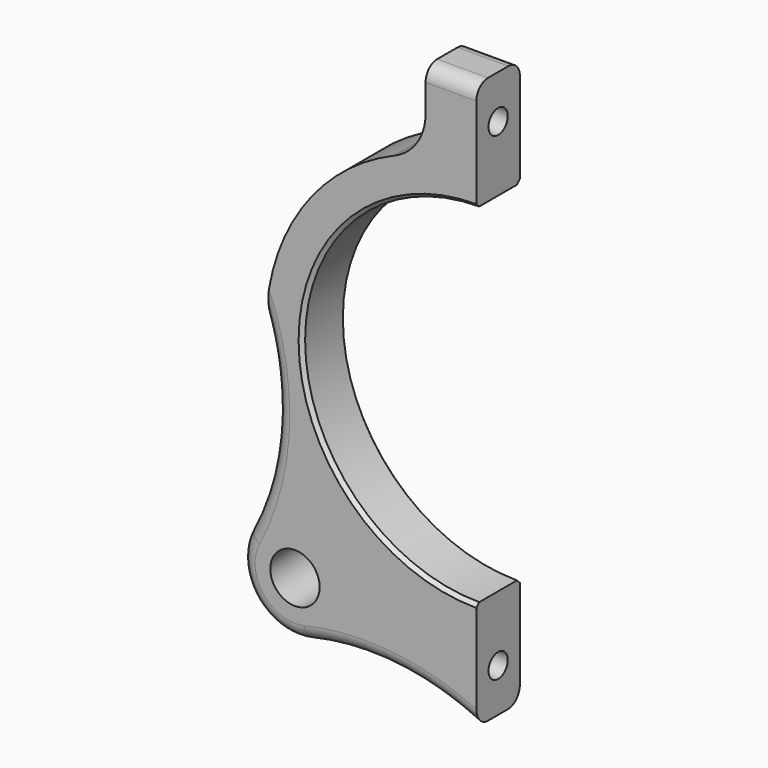
from build123d import *
from build123d import SkipClean  # not in build123d's __all__

# Parameters (mm, degrees)
F1_DEPTH    = 3.75
F3_D        = 3.3
F3_DEPTH    = 12.2
F3_TIP      = 0.9914200214
F4_R        = 2
F5_T4_DEPTH = 7.5
F5_S5_R     = 1.65
F5_T6_DEPTH = 7
F6_SIZE     = 0.5
F8_D        = 6.8


# Not quite as in the source:
# - a fillet or chamfer that OpenCascade refuses, or shapes differently, is made with other operations: its cross-section is extruded or revolved along the edge and cut away or added
# - a feature names something its author has since deleted; it is built from what else it names


with BuildPart() as f1:
    # F0 (on Front) → F1 (new body, symmetric)
    with BuildSketch(Plane.XZ):
        with BuildLine():
            ThreePointArc((0, -24), (-24, 0), (0, 24))
            Line((0, 24), (0, 39))
            Line((0, 39), (-7, 39))
            Line((-7, 39), (-7, 28.1424945589))
            ThreePointArc((-7, 28.1424945589), (-22.8473193176, 17.8605710995), (-29, 0))
            ThreePointArc((-29, 0), (-27.9004726433, -13.0232858743), (-31.6552133192, -25.541946259))
            ThreePointArc((-31.6552133192, -25.541946259), (-30.9284075442, -33.5939072683), (-23.3128108861, -36.3077625094))
            ThreePointArc((-23.3128108861, -36.3077625094), (-11.4240360348, -35.6417318474), (0, -39))
            Line((0, -39), (0, -24))
        make_face()
    extrude(amount=F1_DEPTH, both=True)

    # F3
    with Locations(Plane.YZ):
        with Locations((0, 33), (0, -33)):
            Hole(F3_D / 2, depth=F3_DEPTH)
            with Locations((0, 0, -(F3_DEPTH + F3_TIP / 2))):  # 118° drill point
                Cone(0, F3_D / 2, F3_TIP, mode=Mode.SUBTRACT)

    # F4
    f4_edges = [f1.edges().sort_by_distance(p)[0] for p in [
        (-3.5, 3.75, 39),
        (-3.5, -3.75, 39),
        (-11.424036, 3.75, -35.641732),
        (-11.424036, -3.75, -35.641732),
    ]]
    fillet(f4_edges, radius=F4_R)

    # F5: fillet of radius 7 on 1 edges, made by hand


with BuildPart() as f5_tool2:
    # F5_s3 → F5_t4 (new body)
    with BuildSketch(Plane.XZ.offset(-3.75)):
        with BuildLine():
            ThreePointArc((-11.2777777778, 26.7172552556), (-8.1666666667, 29.2968523148), (-7, 33.1662479036))
            Line((-7, 33.1662479036), (-7, 28.1424945589))
            ThreePointArc((-7, 28.1424945589), (-9.1666306182, 27.5131401899), (-11.2777777778, 26.7172552556))
        make_face()
    extrude(amount=F5_T4_DEPTH)

    # F5_s5 → F5_t6 (cut, symmetric)
    with BuildSketch(Plane.YZ.offset(-9.1)):
        with Locations((0, 33)):
            Circle(F5_S5_R)
    with SkipClean():  # cleaning this boolean's faces spoils the solid; the shape is the same uncleaned
        extrude(amount=F5_T6_DEPTH, both=True, mode=Mode.SUBTRACT)


with BuildPart() as f1_1:
    add(f1.part, clean=False)

    # F5_t1: union F5_tool2
    add(f5_tool2.part)

    # F6
    f6_edges = [f1_1.edges().sort_by_distance(p)[0] for p in [
        (-24, 3.75, 0),
        (-24, -3.75, 0),
    ]]
    chamfer(f6_edges, length=F6_SIZE)

    # F8 (through all)
    with Locations(Plane.XZ.offset(3.75)):
        with Locations((-25, -29)):
            Hole(F8_D / 2)


solid = f1_1.part
